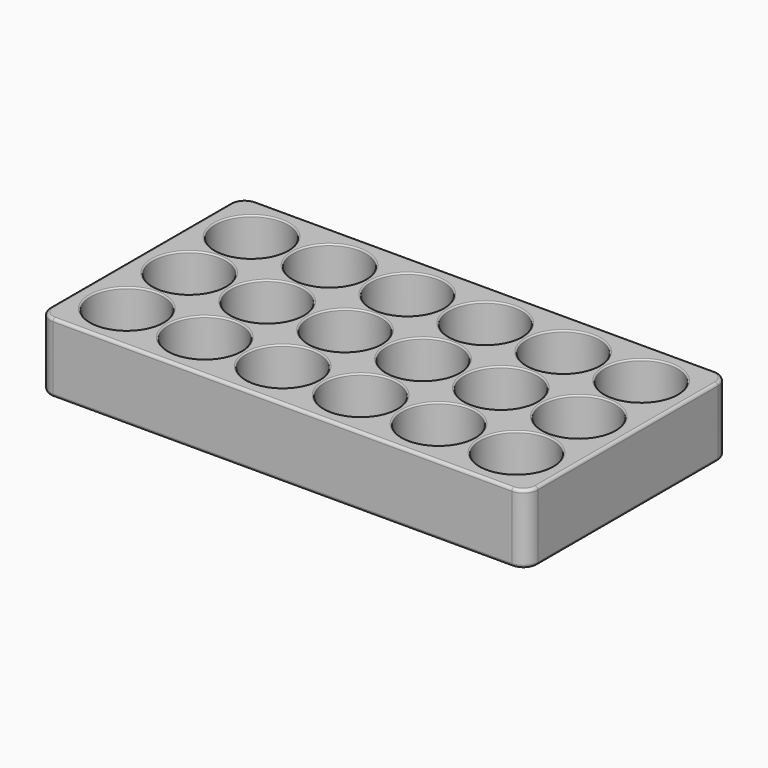
from build123d import *

# Parameters (mm, degrees)
F0_W         = 169
F0_H         = 88
F0_R         = 12.6
F1_DEPTH     = 22
F2_W         = 169
F2_H         = 88
F3_DEPTH     = 2
F4_R         = 1
F5_R         = 0.5
F6_T1_DEPTH  = 24
F6_T4_ANGLE  = 90
F6_T6_ANGLE  = 90
F6_T8_ANGLE  = 90
F6_T10_ANGLE = 90
F6_T12_ANGLE = 90
F6_T14_ANGLE = 90
F6_T16_ANGLE = 90
F6_T18_ANGLE = 90


# Not quite as in the source:
# - a fillet or chamfer that OpenCascade refuses, or shapes differently, is made with other operations: its cross-section is extruded or revolved along the edge and cut away or added


with BuildPart() as f1:
    # F0 (on Top) → F1 (new body)
    with BuildSketch(Plane.XY):
        with Locations((67.5, 27)):
            Rectangle(F0_W, F0_H)
        Circle(F0_R, mode=Mode.SUBTRACT)
        with Locations((27, 0)):
            Circle(F0_R, mode=Mode.SUBTRACT)
        with Locations((54, 0)):
            Circle(F0_R, mode=Mode.SUBTRACT)
        with Locations((81, 0)):
            Circle(F0_R, mode=Mode.SUBTRACT)
        with Locations((108, 0)):
            Circle(F0_R, mode=Mode.SUBTRACT)
        with Locations((135, 0)):
            Circle(F0_R, mode=Mode.SUBTRACT)
        with Locations((0, 27)):
            Circle(F0_R, mode=Mode.SUBTRACT)
        with Locations((27, 27)):
            Circle(F0_R, mode=Mode.SUBTRACT)
        with Locations((54, 27)):
            Circle(F0_R, mode=Mode.SUBTRACT)
        with Locations((0, 54)):
            Circle(F0_R, mode=Mode.SUBTRACT)
        with Locations((27, 54)):
            Circle(F0_R, mode=Mode.SUBTRACT)
        with Locations((54, 54)):
            Circle(F0_R, mode=Mode.SUBTRACT)
        with Locations((81, 27)):
            Circle(F0_R, mode=Mode.SUBTRACT)
        with Locations((108, 27)):
            Circle(F0_R, mode=Mode.SUBTRACT)
        with Locations((135, 27)):
            Circle(F0_R, mode=Mode.SUBTRACT)
        with Locations((81, 54)):
            Circle(F0_R, mode=Mode.SUBTRACT)
        with Locations((108, 54)):
            Circle(F0_R, mode=Mode.SUBTRACT)
        with Locations((135, 54)):
            Circle(F0_R, mode=Mode.SUBTRACT)
    extrude(amount=-F1_DEPTH)

    # F2 (on face) → F3 (join)
    with BuildSketch(Plane(origin=(0, 0, -22), x_dir=(1, 0, 0), z_dir=(0, 0, -1))):
        with Locations((67.5, -27)):
            Rectangle(F2_W, F2_H)
    extrude(amount=F3_DEPTH)

    # F4
    f4_edges = [f1.edges().sort_by_distance(p)[0] for p in [
        (-17, 27, 0),
        (67.5, 71, 0),
        (152, 27, 0),
        (67.5, -17, 0),
        (67.5, 71, -24),
        (152, 27, -24),
        (67.5, -17, -24),
        (-17, 27, -24),
    ]]
    fillet(f4_edges, radius=F4_R)

    # F5
    f5_edges = [f1.edges().sort_by_distance(p)[0] for p in [
        (122.4, 0, 0),
        (-16, 27, 0),
        (67.5, 70, 0),
        (67.5, -16, 0),
        (151, 27, 0),
        (-12.6, 0, 0),
        (14.4, 0, 0),
        (41.4, 0, 0),
        (68.4, 0, 0),
        (95.4, 0, 0),
        (-12.6, 27, 0),
        (14.4, 27, 0),
        (41.4, 27, 0),
        (-12.6, 54, 0),
        (14.4, 54, 0),
        (41.4, 54, 0),
        (68.4, 27, 0),
        (95.4, 27, 0),
        (122.4, 27, 0),
        (68.4, 54, 0),
        (95.4, 54, 0),
        (122.4, 54, 0),
    ]]
    fillet(f5_edges, radius=F5_R)

    # F6: fillet of radius 5 on 4 edges, made by hand

    # F6_s2 → F6_t1 (cut)
    with BuildSketch(Plane.XY.offset(-24)):
        with BuildLine():
            ThreePointArc((-17, 66), (-15.5355339059, 69.5355339059), (-12, 71))
            Line((-12, 71), (-17, 71))
            Line((-17, 71), (-17, 66))
        make_face()
        with BuildLine():
            ThreePointArc((-17, -12), (-15.5355339059, -15.5355339059), (-12, -17))
            Line((-12, -17), (-17, -17))
            Line((-17, -17), (-17, -12))
        make_face()
        with BuildLine():
            ThreePointArc((147, 71), (150.5355339059, 69.5355339059), (152, 66))
            Line((152, 66), (152, 71))
            Line((152, 71), (147, 71))
        make_face()
        with BuildLine():
            ThreePointArc((147, -17), (150.5355339059, -15.5355339059), (152, -12))
            Line((152, -12), (152, -17))
            Line((152, -17), (147, -17))
        make_face()
    extrude(amount=F6_T1_DEPTH, mode=Mode.SUBTRACT)

    # F6_s3 → F6_t4 (revolve, cut)
    with BuildSketch(Plane.YZ.offset(147)):
        with BuildLine():
            ThreePointArc((-16, 0), (-16.7071067812, -0.2928932188), (-17, -1))
            Line((-17, -1), (-17, 0))
            Line((-17, 0), (-16, 0))
        make_face()
    revolve(axis=Axis((147, -12, 0), (0, 0, 1)), revolution_arc=F6_T4_ANGLE, mode=Mode.SUBTRACT)

    # F6_s5 → F6_t6 (revolve, cut)
    with BuildSketch(Plane.XZ.offset(12)):
        with BuildLine():
            ThreePointArc((151, -24), (151.7071067812, -23.7071067812), (152, -23))
            Line((152, -23), (152, -24))
            Line((152, -24), (151, -24))
        make_face()
    revolve(axis=Axis((147, -12, -24), (0, 0, -1)), revolution_arc=F6_T6_ANGLE, mode=Mode.SUBTRACT)

    # F6_s7 → F6_t8 (revolve, cut)
    with BuildSketch(Plane.XZ.offset(-66)):
        with BuildLine():
            ThreePointArc((151, 0), (151.7071067812, -0.2928932188), (152, -1))
            Line((152, -1), (152, 0))
            Line((152, 0), (151, 0))
        make_face()
    revolve(axis=Axis((147, 66, 0), (0, 0, 1)), revolution_arc=F6_T8_ANGLE, mode=Mode.SUBTRACT)

    # F6_s9 → F6_t10 (revolve, cut)
    with BuildSketch(Plane.YZ.offset(147)):
        with BuildLine():
            ThreePointArc((70, -24), (70.7071067812, -23.7071067812), (71, -23))
            Line((71, -23), (71, -24))
            Line((71, -24), (70, -24))
        make_face()
    revolve(axis=Axis((147, 66, -24), (0, 0, -1)), revolution_arc=F6_T10_ANGLE, mode=Mode.SUBTRACT)

    # F6_s11 → F6_t12 (revolve, cut)
    with BuildSketch(Plane.YZ.offset(-12)):
        with BuildLine():
            ThreePointArc((-16, -24), (-16.7071067812, -23.7071067812), (-17, -23))
            Line((-17, -23), (-17, -24))
            Line((-17, -24), (-16, -24))
        make_face()
    revolve(axis=Axis((-12, -12, -24), (0, 0, -1)), revolution_arc=F6_T12_ANGLE, mode=Mode.SUBTRACT)

    # F6_s13 → F6_t14 (revolve, cut)
    with BuildSketch(Plane.XZ.offset(12)):
        with BuildLine():
            ThreePointArc((-16, 0), (-16.7071067812, -0.2928932188), (-17, -1))
            Line((-17, -1), (-17, 0))
            Line((-17, 0), (-16, 0))
        make_face()
    revolve(axis=Axis((-12, -12, 0), (0, 0, 1)), revolution_arc=F6_T14_ANGLE, mode=Mode.SUBTRACT)

    # F6_s15 → F6_t16 (revolve, cut)
    with BuildSketch(Plane.XZ.offset(-66)):
        with BuildLine():
            ThreePointArc((-16, -24), (-16.7071067812, -23.7071067812), (-17, -23))
            Line((-17, -23), (-17, -24))
            Line((-17, -24), (-16, -24))
        make_face()
    revolve(axis=Axis((-12, 66, -24), (0, 0, -1)), revolution_arc=F6_T16_ANGLE, mode=Mode.SUBTRACT)

    # F6_s17 → F6_t18 (revolve, cut)
    with BuildSketch(Plane.YZ.offset(-12)):
        with BuildLine():
            ThreePointArc((70, 0), (70.7071067812, -0.2928932188), (71, -1))
            Line((71, -1), (71, 0))
            Line((71, 0), (70, 0))
        make_face()
    revolve(axis=Axis((-12, 66, 0), (0, 0, 1)), revolution_arc=F6_T18_ANGLE, mode=Mode.SUBTRACT)


solid = f1.part
